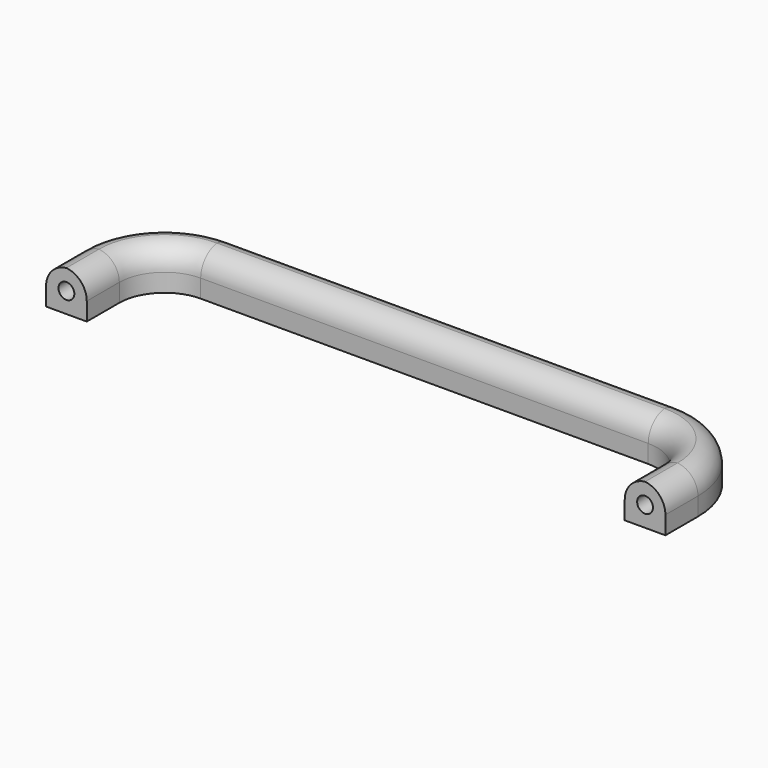
from build123d import *

# Parameters (mm, degrees)
F1_DEPTH     = 9
F2_T1_DEPTH  = 21.5
F2_T3_DEPTH  = 99
F2_T6_ANGLE  = 90
F2_T8_ANGLE  = 90
F2_T10_ANGLE = 90
F2_T12_ANGLE = 90
F3_R         = 1.75
F4_DEPTH     = 13


# Not quite as in the source:
# - a fillet or chamfer that OpenCascade refuses, or shapes differently, is made with other operations: its cross-section is extruded or revolved along the edge and cut away or added


with BuildPart() as f1:
    # F0 (on Top) → F1 (new body)
    with BuildSketch(Plane.XY):
        with BuildLine():
            Line((0, 9), (0, 0))
            Line((0, 0), (9, 0))
            Line((9, 0), (9, 9))
            ThreePointArc((9, 9), (11.9289321881, 16.0710678119), (19, 19))
            Line((19, 19), (118, 19))
            ThreePointArc((118, 19), (125.0710678119, 16.0710678119), (128, 9))
            Line((128, 9), (128, 0))
            Line((128, 0), (137, 0))
            Line((137, 0), (137, 9))
            ThreePointArc((137, 9), (131.4350288425, 22.4350288425), (118, 28))
            Line((118, 28), (19, 28))
            ThreePointArc((19, 28), (5.5649711575, 22.4350288425), (0, 9))
        make_face()
    extrude(amount=F1_DEPTH)

    # F2: fillet of radius 5 on 7 edges, made by hand

    # F2_s2 → F2_t1 (cut)
    with BuildSketch(Plane.XZ.offset(-9)):
        with BuildLine():
            ThreePointArc((0, 4), (1.4644660941, 7.5355339059), (5, 9))
            Line((5, 9), (0, 9))
            Line((0, 9), (0, 4))
        make_face()
        with BuildLine():
            ThreePointArc((137, 4), (135.5355339059, 7.5355339059), (132, 9))
            Line((132, 9), (137, 9))
            Line((137, 9), (137, 4))
        make_face()
        with BuildLine():
            ThreePointArc((128, 4), (129.4644660941, 7.5355339059), (133, 9))
            Line((133, 9), (128, 9))
            Line((128, 9), (128, 4))
        make_face()
        with BuildLine():
            ThreePointArc((9, 4), (7.5355339059, 7.5355339059), (4, 9))
            Line((4, 9), (9, 9))
            Line((9, 9), (9, 4))
        make_face()
    extrude(amount=F2_T1_DEPTH, mode=Mode.SUBTRACT)

    # F2_s4 → F2_t3 (cut)
    with BuildSketch(Plane.YZ.offset(19)):
        with BuildLine():
            ThreePointArc((28, 4), (26.5355339059, 7.5355339059), (23, 9))
            Line((23, 9), (28, 9))
            Line((28, 9), (28, 4))
        make_face()
        with BuildLine():
            ThreePointArc((19, 4), (20.4644660941, 7.5355339059), (24, 9))
            Line((24, 9), (19, 9))
            Line((19, 9), (19, 4))
        make_face()
    extrude(amount=F2_T3_DEPTH, mode=Mode.SUBTRACT)

    # F2_s5 → F2_t6 (revolve, cut)
    with BuildSketch(Plane.YZ.offset(19)):
        with BuildLine():
            ThreePointArc((28, 4), (26.5355339059, 7.5355339059), (23, 9))
            Line((23, 9), (28, 9))
            Line((28, 9), (28, 4))
        make_face()
    revolve(axis=Axis((19, 9, 9), (0, 0, 1)), revolution_arc=F2_T6_ANGLE, mode=Mode.SUBTRACT)

    # F2_s7 → F2_t8 (revolve, cut)
    with BuildSketch(Plane.XZ.offset(-9)):
        with BuildLine():
            ThreePointArc((137, 4), (135.5355339059, 7.5355339059), (132, 9))
            Line((132, 9), (137, 9))
            Line((137, 9), (137, 4))
        make_face()
    revolve(axis=Axis((118, 9, 9), (0, 0, 1)), revolution_arc=F2_T8_ANGLE, mode=Mode.SUBTRACT)

    # F2_s9 → F2_t10 (revolve, cut)
    with BuildSketch(Plane.YZ.offset(118)):
        with BuildLine():
            ThreePointArc((19, 4), (20.4644660941, 7.5355339059), (24, 9))
            Line((24, 9), (19, 9))
            Line((19, 9), (19, 4))
        make_face()
    revolve(axis=Axis((118, 9, 9), (0, 0, -1)), revolution_arc=F2_T10_ANGLE, mode=Mode.SUBTRACT)

    # F2_s11 → F2_t12 (revolve, cut)
    with BuildSketch(Plane.XZ.offset(-9)):
        with BuildLine():
            ThreePointArc((9, 4), (7.5355339059, 7.5355339059), (4, 9))
            Line((4, 9), (9, 9))
            Line((9, 9), (9, 4))
        make_face()
    revolve(axis=Axis((19, 9, 9), (0, 0, -1)), revolution_arc=F2_T12_ANGLE, mode=Mode.SUBTRACT)

    # F3 (on face) → F4 (cut)
    with BuildSketch(Plane.XZ):
        with Locations((4.5, 4.5)):
            Circle(F3_R)
        with Locations((132.5, 4.5)):
            Circle(F3_R)
    extrude(amount=-F4_DEPTH, mode=Mode.SUBTRACT)


solid = f1.part
